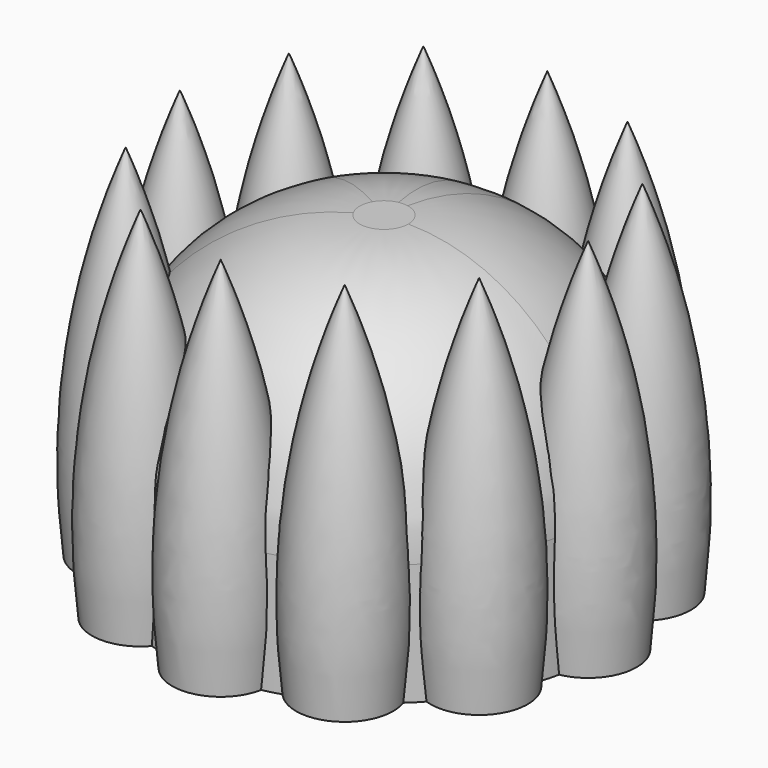
from build123d import *

# Parameters (mm, degrees)
F1_DEPTH  = 16.51
F2_R      = 10.16
F3_T      = -1.016
F7_COUNT  = 12
F8_R      = 1.397
F9_DEPTH  = 8.89
F10_R     = 1.016
F12_COUNT = 12


# Not quite as in the source:
# - a feature names something its author has since deleted; it is built from what else it names


with BuildPart() as f1:
    # F0 (on Top) → F1 (new body)
    with BuildSketch(Plane.XY):
        with BuildLine():
            ThreePointArc((-9.9705175686, -5.5887099955), (2.8880689215, -11.0591119854), (11.43, 0))
            ThreePointArc((11.43, 0), (8.8094257887, 7.2827822481), (2.1493495585, 11.2260944444))
            ThreePointArc((2.1493495585, 11.2260944444), (0, 9.271), (-2.1493495585, 11.2260944444))
            ThreePointArc((-2.1493495585, 11.2260944444), (-6.6833988846, 9.2723826145), (-9.9705175686, 5.5887099955))
            Line((-9.9705175686, 5.5887099955), (0, 0))
            Line((0, 0), (-9.9705175686, -5.5887099955))
        make_face()
        with BuildLine():
            ThreePointArc((-9.9705175686, 5.5887099955), (-11.43, 0), (-9.9705175686, -5.5887099955))
            Line((-9.9705175686, -5.5887099955), (0, 0))
            Line((0, 0), (-9.9705175686, 5.5887099955))
        make_face()
        with BuildLine():
            ThreePointArc((-2.1493495585, 11.2260944444), (0, 9.271), (2.1493495585, 11.2260944444))
            ThreePointArc((2.1493495585, 11.2260944444), (0, 11.43), (-2.1493495585, 11.2260944444))
        make_face()
    extrude(amount=F1_DEPTH)

    # F2
    f2_edges = [f1.edges().sort_by_distance(p)[0] for p in [
        (-2.14935, -11.226094, 16.51),
    ]]
    fillet(f2_edges, radius=F2_R)

    # F3
    f3_openings = [f1.faces().sort_by_distance(p)[0] for p in [
        (0, 0, 0),
    ]]
    offset(amount=F3_T, openings=f3_openings)


with BuildPart() as f5:
    # F4 (on Front) → F5 (revolve)
    with BuildSketch(Plane.XZ):
        with BuildLine():
            Line((0, 18.796), (0, 0))
            Line((0, 0), (2.54, 0))
            ThreePointArc((2.54, 0), (2.4495974066, 9.5574050549), (0, 18.796))
        make_face()
    revolve(axis=Axis((0, 0, 20.1927059578), (0, 0, 1)))


with BuildPart() as f5_1:
    # F6: moved
    add(f5.part.moved(Location((10.668, 0, 0))))


with BuildPart() as f7_1:
    # F7: instance of F5
    add(f5_1.part.rotate(Axis((0, 0, 0), (0, 0, 1)), 1 * 360 / F7_COUNT))


with BuildPart() as f7_2:
    # F7: instance of F5
    add(f5_1.part.rotate(Axis((0, 0, 0), (0, 0, 1)), 2 * 360 / F7_COUNT))


with BuildPart() as f7_3:
    # F7: instance of F5
    add(f5_1.part.rotate(Axis((0, 0, 0), (0, 0, 1)), 3 * 360 / F7_COUNT))


with BuildPart() as f7_4:
    # F7: instance of F5
    add(f5_1.part.rotate(Axis((0, 0, 0), (0, 0, 1)), 4 * 360 / F7_COUNT))


with BuildPart() as f7_5:
    # F7: instance of F5
    add(f5_1.part.rotate(Axis((0, 0, 0), (0, 0, 1)), 5 * 360 / F7_COUNT))


with BuildPart() as f7_6:
    # F7: instance of F5
    add(f5_1.part.rotate(Axis((0, 0, 0), (0, 0, 1)), 6 * 360 / F7_COUNT))


with BuildPart() as f7_7:
    # F7: instance of F5
    add(f5_1.part.rotate(Axis((0, 0, 0), (0, 0, 1)), 7 * 360 / F7_COUNT))


with BuildPart() as f7_8:
    # F7: instance of F5
    add(f5_1.part.rotate(Axis((0, 0, 0), (0, 0, 1)), 8 * 360 / F7_COUNT))


with BuildPart() as f7_9:
    # F7: instance of F5
    add(f5_1.part.rotate(Axis((0, 0, 0), (0, 0, 1)), 9 * 360 / F7_COUNT))


with BuildPart() as f7_10:
    # F7: instance of F5
    add(f5_1.part.rotate(Axis((0, 0, 0), (0, 0, 1)), 10 * 360 / F7_COUNT))


with BuildPart() as f7_11:
    # F7: instance of F5
    add(f5_1.part.rotate(Axis((0, 0, 0), (0, 0, 1)), 11 * 360 / F7_COUNT))


with BuildPart() as f9:
    # F8 (on Top) → F9 (new body, symmetric)
    with BuildSketch(Plane.XY):
        Circle(F8_R)
    extrude(amount=F9_DEPTH, both=True)

    # F10
    f10_edges = [f9.edges().sort_by_distance(p)[0] for p in [
        (-1.397, 0, 8.89),
    ]]
    fillet(f10_edges, radius=F10_R)


with BuildPart() as f9_1:
    # F11: moved
    add(f9.part.moved(Location((10.668, 0, 0))))


with BuildPart() as f12_1:
    # F12: instance of F9
    add(f9_1.part.rotate(Axis((0, 0, 0), (0, 0, 1)), 1 * 360 / F12_COUNT))


with BuildPart() as f12_2:
    # F12: instance of F9
    add(f9_1.part.rotate(Axis((0, 0, 0), (0, 0, 1)), 2 * 360 / F12_COUNT))


with BuildPart() as f12_3:
    # F12: instance of F9
    add(f9_1.part.rotate(Axis((0, 0, 0), (0, 0, 1)), 3 * 360 / F12_COUNT))


with BuildPart() as f12_4:
    # F12: instance of F9
    add(f9_1.part.rotate(Axis((0, 0, 0), (0, 0, 1)), 4 * 360 / F12_COUNT))


with BuildPart() as f12_5:
    # F12: instance of F9
    add(f9_1.part.rotate(Axis((0, 0, 0), (0, 0, 1)), 5 * 360 / F12_COUNT))


with BuildPart() as f12_6:
    # F12: instance of F9
    add(f9_1.part.rotate(Axis((0, 0, 0), (0, 0, 1)), 6 * 360 / F12_COUNT))


with BuildPart() as f12_7:
    # F12: instance of F9
    add(f9_1.part.rotate(Axis((0, 0, 0), (0, 0, 1)), 7 * 360 / F12_COUNT))


with BuildPart() as f12_8:
    # F12: instance of F9
    add(f9_1.part.rotate(Axis((0, 0, 0), (0, 0, 1)), 8 * 360 / F12_COUNT))


with BuildPart() as f12_9:
    # F12: instance of F9
    add(f9_1.part.rotate(Axis((0, 0, 0), (0, 0, 1)), 9 * 360 / F12_COUNT))


with BuildPart() as f12_10:
    # F12: instance of F9
    add(f9_1.part.rotate(Axis((0, 0, 0), (0, 0, 1)), 10 * 360 / F12_COUNT))


with BuildPart() as f12_11:
    # F12: instance of F9
    add(f9_1.part.rotate(Axis((0, 0, 0), (0, 0, 1)), 11 * 360 / F12_COUNT))


with BuildPart() as f1_1:
    add(f1.part)

    # F13: cut F12_9, F12_10, F12_11, F9, F12_1, F12_2, F12_3, F12_4, F12_5, F12_6, F12_7, F12_8
    add(f12_9.part, mode=Mode.SUBTRACT)
    add(f12_10.part, mode=Mode.SUBTRACT)
    add(f12_11.part, mode=Mode.SUBTRACT)
    add(f9_1.part, mode=Mode.SUBTRACT)
    add(f12_1.part, mode=Mode.SUBTRACT)
    add(f12_2.part, mode=Mode.SUBTRACT)
    add(f12_3.part, mode=Mode.SUBTRACT)
    add(f12_4.part, mode=Mode.SUBTRACT)
    add(f12_5.part, mode=Mode.SUBTRACT)
    add(f12_6.part, mode=Mode.SUBTRACT)
    add(f12_7.part, mode=Mode.SUBTRACT)
    add(f12_8.part, mode=Mode.SUBTRACT)


with BuildPart() as f7_3_1:
    add(f7_3.part)

    # F13: cut F12_9, F12_10, F12_11, F9, F12_1, F12_2, F12_3, F12_4, F12_5, F12_6, F12_7, F12_8
    add(f12_9.part, mode=Mode.SUBTRACT)
    add(f12_10.part, mode=Mode.SUBTRACT)
    add(f12_11.part, mode=Mode.SUBTRACT)
    add(f9_1.part, mode=Mode.SUBTRACT)
    add(f12_1.part, mode=Mode.SUBTRACT)
    add(f12_2.part, mode=Mode.SUBTRACT)
    add(f12_3.part, mode=Mode.SUBTRACT)
    add(f12_4.part, mode=Mode.SUBTRACT)
    add(f12_5.part, mode=Mode.SUBTRACT)
    add(f12_6.part, mode=Mode.SUBTRACT)
    add(f12_7.part, mode=Mode.SUBTRACT)
    add(f12_8.part, mode=Mode.SUBTRACT)


with BuildPart() as f7_2_1:
    add(f7_2.part)

    # F13: cut F12_9, F12_10, F12_11, F9, F12_1, F12_2, F12_3, F12_4, F12_5, F12_6, F12_7, F12_8
    add(f12_9.part, mode=Mode.SUBTRACT)
    add(f12_10.part, mode=Mode.SUBTRACT)
    add(f12_11.part, mode=Mode.SUBTRACT)
    add(f9_1.part, mode=Mode.SUBTRACT)
    add(f12_1.part, mode=Mode.SUBTRACT)
    add(f12_2.part, mode=Mode.SUBTRACT)
    add(f12_3.part, mode=Mode.SUBTRACT)
    add(f12_4.part, mode=Mode.SUBTRACT)
    add(f12_5.part, mode=Mode.SUBTRACT)
    add(f12_6.part, mode=Mode.SUBTRACT)
    add(f12_7.part, mode=Mode.SUBTRACT)
    add(f12_8.part, mode=Mode.SUBTRACT)


with BuildPart() as f7_1_1:
    add(f7_1.part)

    # F13: cut F12_9, F12_10, F12_11, F9, F12_1, F12_2, F12_3, F12_4, F12_5, F12_6, F12_7, F12_8
    add(f12_9.part, mode=Mode.SUBTRACT)
    add(f12_10.part, mode=Mode.SUBTRACT)
    add(f12_11.part, mode=Mode.SUBTRACT)
    add(f9_1.part, mode=Mode.SUBTRACT)
    add(f12_1.part, mode=Mode.SUBTRACT)
    add(f12_2.part, mode=Mode.SUBTRACT)
    add(f12_3.part, mode=Mode.SUBTRACT)
    add(f12_4.part, mode=Mode.SUBTRACT)
    add(f12_5.part, mode=Mode.SUBTRACT)
    add(f12_6.part, mode=Mode.SUBTRACT)
    add(f12_7.part, mode=Mode.SUBTRACT)
    add(f12_8.part, mode=Mode.SUBTRACT)


with BuildPart() as f5_2:
    add(f5_1.part)

    # F13: cut F12_9, F12_10, F12_11, F9, F12_1, F12_2, F12_3, F12_4, F12_5, F12_6, F12_7, F12_8
    add(f12_9.part, mode=Mode.SUBTRACT)
    add(f12_10.part, mode=Mode.SUBTRACT)
    add(f12_11.part, mode=Mode.SUBTRACT)
    add(f9_1.part, mode=Mode.SUBTRACT)
    add(f12_1.part, mode=Mode.SUBTRACT)
    add(f12_2.part, mode=Mode.SUBTRACT)
    add(f12_3.part, mode=Mode.SUBTRACT)
    add(f12_4.part, mode=Mode.SUBTRACT)
    add(f12_5.part, mode=Mode.SUBTRACT)
    add(f12_6.part, mode=Mode.SUBTRACT)
    add(f12_7.part, mode=Mode.SUBTRACT)
    add(f12_8.part, mode=Mode.SUBTRACT)


with BuildPart() as f7_11_1:
    add(f7_11.part)

    # F13: cut F12_9, F12_10, F12_11, F9, F12_1, F12_2, F12_3, F12_4, F12_5, F12_6, F12_7, F12_8
    add(f12_9.part, mode=Mode.SUBTRACT)
    add(f12_10.part, mode=Mode.SUBTRACT)
    add(f12_11.part, mode=Mode.SUBTRACT)
    add(f9_1.part, mode=Mode.SUBTRACT)
    add(f12_1.part, mode=Mode.SUBTRACT)
    add(f12_2.part, mode=Mode.SUBTRACT)
    add(f12_3.part, mode=Mode.SUBTRACT)
    add(f12_4.part, mode=Mode.SUBTRACT)
    add(f12_5.part, mode=Mode.SUBTRACT)
    add(f12_6.part, mode=Mode.SUBTRACT)
    add(f12_7.part, mode=Mode.SUBTRACT)
    add(f12_8.part, mode=Mode.SUBTRACT)


with BuildPart() as f7_10_1:
    add(f7_10.part)

    # F13: cut F12_9, F12_10, F12_11, F9, F12_1, F12_2, F12_3, F12_4, F12_5, F12_6, F12_7, F12_8
    add(f12_9.part, mode=Mode.SUBTRACT)
    add(f12_10.part, mode=Mode.SUBTRACT)
    add(f12_11.part, mode=Mode.SUBTRACT)
    add(f9_1.part, mode=Mode.SUBTRACT)
    add(f12_1.part, mode=Mode.SUBTRACT)
    add(f12_2.part, mode=Mode.SUBTRACT)
    add(f12_3.part, mode=Mode.SUBTRACT)
    add(f12_4.part, mode=Mode.SUBTRACT)
    add(f12_5.part, mode=Mode.SUBTRACT)
    add(f12_6.part, mode=Mode.SUBTRACT)
    add(f12_7.part, mode=Mode.SUBTRACT)
    add(f12_8.part, mode=Mode.SUBTRACT)


with BuildPart() as f7_9_1:
    add(f7_9.part)

    # F13: cut F12_9, F12_10, F12_11, F9, F12_1, F12_2, F12_3, F12_4, F12_5, F12_6, F12_7, F12_8
    add(f12_9.part, mode=Mode.SUBTRACT)
    add(f12_10.part, mode=Mode.SUBTRACT)
    add(f12_11.part, mode=Mode.SUBTRACT)
    add(f9_1.part, mode=Mode.SUBTRACT)
    add(f12_1.part, mode=Mode.SUBTRACT)
    add(f12_2.part, mode=Mode.SUBTRACT)
    add(f12_3.part, mode=Mode.SUBTRACT)
    add(f12_4.part, mode=Mode.SUBTRACT)
    add(f12_5.part, mode=Mode.SUBTRACT)
    add(f12_6.part, mode=Mode.SUBTRACT)
    add(f12_7.part, mode=Mode.SUBTRACT)
    add(f12_8.part, mode=Mode.SUBTRACT)


with BuildPart() as f7_8_1:
    add(f7_8.part)

    # F13: cut F12_9, F12_10, F12_11, F9, F12_1, F12_2, F12_3, F12_4, F12_5, F12_6, F12_7, F12_8
    add(f12_9.part, mode=Mode.SUBTRACT)
    add(f12_10.part, mode=Mode.SUBTRACT)
    add(f12_11.part, mode=Mode.SUBTRACT)
    add(f9_1.part, mode=Mode.SUBTRACT)
    add(f12_1.part, mode=Mode.SUBTRACT)
    add(f12_2.part, mode=Mode.SUBTRACT)
    add(f12_3.part, mode=Mode.SUBTRACT)
    add(f12_4.part, mode=Mode.SUBTRACT)
    add(f12_5.part, mode=Mode.SUBTRACT)
    add(f12_6.part, mode=Mode.SUBTRACT)
    add(f12_7.part, mode=Mode.SUBTRACT)
    add(f12_8.part, mode=Mode.SUBTRACT)


with BuildPart() as f7_7_1:
    add(f7_7.part)

    # F13: cut F12_9, F12_10, F12_11, F9, F12_1, F12_2, F12_3, F12_4, F12_5, F12_6, F12_7, F12_8
    add(f12_9.part, mode=Mode.SUBTRACT)
    add(f12_10.part, mode=Mode.SUBTRACT)
    add(f12_11.part, mode=Mode.SUBTRACT)
    add(f9_1.part, mode=Mode.SUBTRACT)
    add(f12_1.part, mode=Mode.SUBTRACT)
    add(f12_2.part, mode=Mode.SUBTRACT)
    add(f12_3.part, mode=Mode.SUBTRACT)
    add(f12_4.part, mode=Mode.SUBTRACT)
    add(f12_5.part, mode=Mode.SUBTRACT)
    add(f12_6.part, mode=Mode.SUBTRACT)
    add(f12_7.part, mode=Mode.SUBTRACT)
    add(f12_8.part, mode=Mode.SUBTRACT)


with BuildPart() as f7_6_1:
    add(f7_6.part)

    # F13: cut F12_9, F12_10, F12_11, F9, F12_1, F12_2, F12_3, F12_4, F12_5, F12_6, F12_7, F12_8
    add(f12_9.part, mode=Mode.SUBTRACT)
    add(f12_10.part, mode=Mode.SUBTRACT)
    add(f12_11.part, mode=Mode.SUBTRACT)
    add(f9_1.part, mode=Mode.SUBTRACT)
    add(f12_1.part, mode=Mode.SUBTRACT)
    add(f12_2.part, mode=Mode.SUBTRACT)
    add(f12_3.part, mode=Mode.SUBTRACT)
    add(f12_4.part, mode=Mode.SUBTRACT)
    add(f12_5.part, mode=Mode.SUBTRACT)
    add(f12_6.part, mode=Mode.SUBTRACT)
    add(f12_7.part, mode=Mode.SUBTRACT)
    add(f12_8.part, mode=Mode.SUBTRACT)


with BuildPart() as f7_5_1:
    add(f7_5.part)

    # F13: cut F12_9, F12_10, F12_11, F9, F12_1, F12_2, F12_3, F12_4, F12_5, F12_6, F12_7, F12_8
    add(f12_9.part, mode=Mode.SUBTRACT)
    add(f12_10.part, mode=Mode.SUBTRACT)
    add(f12_11.part, mode=Mode.SUBTRACT)
    add(f9_1.part, mode=Mode.SUBTRACT)
    add(f12_1.part, mode=Mode.SUBTRACT)
    add(f12_2.part, mode=Mode.SUBTRACT)
    add(f12_3.part, mode=Mode.SUBTRACT)
    add(f12_4.part, mode=Mode.SUBTRACT)
    add(f12_5.part, mode=Mode.SUBTRACT)
    add(f12_6.part, mode=Mode.SUBTRACT)
    add(f12_7.part, mode=Mode.SUBTRACT)
    add(f12_8.part, mode=Mode.SUBTRACT)


with BuildPart() as f7_4_1:
    add(f7_4.part)

    # F13: cut F12_9, F12_10, F12_11, F9, F12_1, F12_2, F12_3, F12_4, F12_5, F12_6, F12_7, F12_8
    add(f12_9.part, mode=Mode.SUBTRACT)
    add(f12_10.part, mode=Mode.SUBTRACT)
    add(f12_11.part, mode=Mode.SUBTRACT)
    add(f9_1.part, mode=Mode.SUBTRACT)
    add(f12_1.part, mode=Mode.SUBTRACT)
    add(f12_2.part, mode=Mode.SUBTRACT)
    add(f12_3.part, mode=Mode.SUBTRACT)
    add(f12_4.part, mode=Mode.SUBTRACT)
    add(f12_5.part, mode=Mode.SUBTRACT)
    add(f12_6.part, mode=Mode.SUBTRACT)
    add(f12_7.part, mode=Mode.SUBTRACT)
    add(f12_8.part, mode=Mode.SUBTRACT)


solid = Compound([f1_1.part, f7_3_1.part, f7_2_1.part, f7_1_1.part, f5_2.part, f7_11_1.part, f7_10_1.part, f7_9_1.part, f7_8_1.part, f7_7_1.part, f7_6_1.part, f7_5_1.part, f7_4_1.part])
